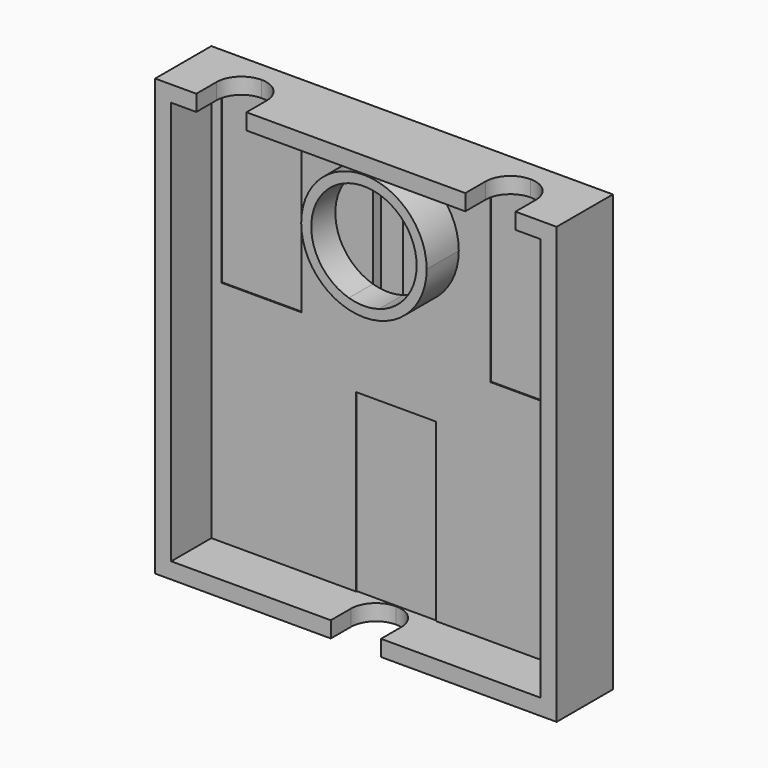
from build123d import *

# Parameters (mm, degrees)
F0_W      = 40
F0_H      = 43.4234265382
F1_DEPTH  = 2
F2_W      = 40
F2_H      = 43.4234265382
F2_W_2    = 36.8
F2_H_2    = 40.2234265382
F3_DEPTH  = 5
F5_DEPTH  = 1.6
F7_DEPTH  = 1
F8_DEPTH  = 4
F9_DEPTH  = 1
F11_DEPTH = 1.6
F13_DEPTH = 0.1


with BuildPart() as f1:
    # F0 (on Front) → F1 (new body)
    with BuildSketch(Plane.XZ):
        with Locations((-15.7519546337, 17.2915523872)):
            Rectangle(F0_W, F0_H)
    extrude(amount=F1_DEPTH)

    # F2 (on face) → F3 (join)
    with BuildSketch(Plane.XZ.offset(2)):
        with Locations((-15.7519546337, 17.2915523872)):
            Rectangle(F2_W, F2_H)
        with Locations((-15.7519546337, 17.2915523872)):
            Rectangle(F2_W_2, F2_H_2, mode=Mode.SUBTRACT)
    extrude(amount=F3_DEPTH)

    # F4 (on face) → F5 (cut, through all)
    with BuildSketch(Plane(origin=(0, 0, 37.4032656563), x_dir=(1, 0, 0), z_dir=(0, 0, -1))):
        with BuildLine():
            ThreePointArc((-4.8519546337, 4.5), (-4.1197215867, 2.732233047), (-2.3519546337, 2))
            ThreePointArc((-2.3519546337, 2), (-0.5841876808, 2.732233047), (0.1480453663, 4.5))
            ThreePointArc((0.1480453663, 4.5), (-0.5841876808, 6.267766953), (-2.3519546337, 7))
            ThreePointArc((-2.3519546337, 7), (-4.1197215867, 6.267766953), (-4.8519546337, 4.5))
        make_face()
        with BuildLine():
            ThreePointArc((-29.1519546337, 2), (-27.3841876808, 2.732233047), (-26.6519546337, 4.5))
            ThreePointArc((-26.6519546337, 4.5), (-27.3841876808, 6.267766953), (-29.1519546337, 7))
            ThreePointArc((-29.1519546337, 7), (-30.9197215867, 6.267766953), (-31.6519546337, 4.5))
            ThreePointArc((-31.6519546337, 4.5), (-30.9197215867, 2.732233047), (-29.1519546337, 2))
        make_face()
        with BuildLine():
            ThreePointArc((-29.1519546337, 7), (-27.3841876808, 6.267766953), (-26.6519546337, 4.5))
            Line((-26.6519546337, 4.5), (-26.6519546337, 7))
            Line((-26.6519546337, 7), (-29.1519546337, 7))
        make_face()
        with BuildLine():
            ThreePointArc((-31.6519546337, 4.5), (-30.9197215867, 6.267766953), (-29.1519546337, 7))
            Line((-29.1519546337, 7), (-31.6519546337, 7))
            Line((-31.6519546337, 7), (-31.6519546337, 4.5))
        make_face()
        with BuildLine():
            Line((-2.3519546337, 7), (-4.8519546337, 7))
            Line((-4.8519546337, 7), (-4.8519546337, 4.5))
            ThreePointArc((-4.8519546337, 4.5), (-4.1197215867, 6.267766953), (-2.3519546337, 7))
        make_face()
        with BuildLine():
            ThreePointArc((-2.3519546337, 7), (-0.5841876808, 6.267766953), (0.1480453663, 4.5))
            Line((0.1480453663, 4.5), (0.1480453663, 7))
            Line((0.1480453663, 7), (-2.3519546337, 7))
        make_face()
    extrude(amount=-F5_DEPTH, mode=Mode.SUBTRACT)

    # F6 (on face) → F7 (join)
    with BuildSketch(Plane.XZ.offset(2)):
        with BuildLine():
            Line((-17.2519546337, 25.3721127069), (-17.2519546337, 35.4344186057))
            ThreePointArc((-17.2519546337, 35.4344186057), (-21.0019546337, 30.4032656563), (-17.2519546337, 25.3721127069))
        make_face()
        with BuildLine():
            ThreePointArc((-14.2519546337, 25.3721127069), (-11.5425900736, 27.2657905568), (-10.5019546337, 30.4032656563))
            ThreePointArc((-10.5019546337, 30.4032656563), (-11.5425900736, 33.5407407558), (-14.2519546337, 35.4344186057))
            Line((-14.2519546337, 35.4344186057), (-14.2519546337, 25.3721127069))
        make_face()
    extrude(amount=F7_DEPTH)

    # F6 (on face) → F8 (join)
    with BuildSketch(Plane.XZ.offset(2)):
        with BuildLine():
            ThreePointArc((-14.2519546337, 35.4344186057), (-11.5425900736, 33.5407407558), (-10.5019546337, 30.4032656563))
            ThreePointArc((-10.5019546337, 30.4032656563), (-11.5425900736, 27.2657905568), (-14.2519546337, 25.3721127069))
            Line((-14.2519546337, 25.3721127069), (-14.2519546337, 24.3359351065))
            ThreePointArc((-14.2519546337, 24.3359351065), (-10.8306997125, 26.5505069044), (-9.5019546337, 30.4032656563))
            ThreePointArc((-9.5019546337, 30.4032656563), (-10.8306997125, 34.2560244081), (-14.2519546337, 36.470596206))
            Line((-14.2519546337, 36.470596206), (-14.2519546337, 35.4344186057))
        make_face()
        with BuildLine():
            ThreePointArc((-17.2519546337, 35.4344186057), (-15.7519546337, 35.6532656563), (-14.2519546337, 35.4344186057))
            Line((-14.2519546337, 35.4344186057), (-14.2519546337, 36.470596206))
            ThreePointArc((-14.2519546337, 36.470596206), (-15.7519546337, 36.6532656563), (-17.2519546337, 36.470596206))
            Line((-17.2519546337, 36.470596206), (-17.2519546337, 35.4344186057))
        make_face()
        with BuildLine():
            Line((-14.2519546337, 24.3359351065), (-14.2519546337, 25.3721127069))
            ThreePointArc((-14.2519546337, 25.3721127069), (-15.7519546337, 25.1532656563), (-17.2519546337, 25.3721127069))
            Line((-17.2519546337, 25.3721127069), (-17.2519546337, 24.3359351065))
            ThreePointArc((-17.2519546337, 24.3359351065), (-15.7519546337, 24.1532656563), (-14.2519546337, 24.3359351065))
        make_face()
        with BuildLine():
            ThreePointArc((-17.2519546337, 25.3721127069), (-21.0019546337, 30.4032656563), (-17.2519546337, 35.4344186057))
            Line((-17.2519546337, 35.4344186057), (-17.2519546337, 36.470596206))
            ThreePointArc((-17.2519546337, 36.470596206), (-22.0019546337, 30.4032656563), (-17.2519546337, 24.3359351065))
            Line((-17.2519546337, 24.3359351065), (-17.2519546337, 25.3721127069))
        make_face()
    extrude(amount=F8_DEPTH)

    # F6 (on face) → F9 (cut)
    with BuildSketch(Plane.XZ.offset(2)):
        with BuildLine():
            ThreePointArc((-17.2519546337, 35.4344186057), (-15.7519546337, 35.6532656563), (-14.2519546337, 35.4344186057))
            Line((-14.2519546337, 35.4344186057), (-14.2519546337, 36.470596206))
            ThreePointArc((-14.2519546337, 36.470596206), (-15.7519546337, 36.6532656563), (-17.2519546337, 36.470596206))
            Line((-17.2519546337, 36.470596206), (-17.2519546337, 35.4344186057))
        make_face()
        with BuildLine():
            Line((-14.2519546337, 24.3359351065), (-14.2519546337, 25.3721127069))
            ThreePointArc((-14.2519546337, 25.3721127069), (-15.7519546337, 25.1532656563), (-17.2519546337, 25.3721127069))
            Line((-17.2519546337, 25.3721127069), (-17.2519546337, 24.3359351065))
            ThreePointArc((-17.2519546337, 24.3359351065), (-15.7519546337, 24.1532656563), (-14.2519546337, 24.3359351065))
        make_face()
    extrude(amount=F9_DEPTH, mode=Mode.SUBTRACT)

    # F10 (on face) → F11 (cut, through all)
    with BuildSketch(Plane.XY.offset(-2.8201608819)):
        with BuildLine():
            Line((-13.2519546337, -7), (-13.2519546337, -4.5))
            ThreePointArc((-13.2519546337, -4.5), (-13.9841876808, -6.267766953), (-15.7519546337, -7))
            Line((-15.7519546337, -7), (-13.2519546337, -7))
        make_face()
        with BuildLine():
            ThreePointArc((-15.7519546337, -7), (-13.9841876808, -6.267766953), (-13.2519546337, -4.5))
            ThreePointArc((-13.2519546337, -4.5), (-13.984187679, -2.7322330488), (-15.7519546286, -2))
            ThreePointArc((-15.7519546286, -2), (-17.5197215849, -2.7322330452), (-18.2519546337, -4.5))
            ThreePointArc((-18.2519546337, -4.5), (-17.5197215867, -6.267766953), (-15.7519546337, -7))
        make_face()
        with BuildLine():
            Line((-18.2519546337, -7), (-15.7519546337, -7))
            ThreePointArc((-15.7519546337, -7), (-17.5197215867, -6.267766953), (-18.2519546337, -4.5))
            Line((-18.2519546337, -4.5), (-18.2519546337, -7))
        make_face()
    extrude(amount=-F11_DEPTH, mode=Mode.SUBTRACT)

    # F12 (on face) → F13 (cut)
    with BuildSketch(Plane.XZ.offset(2)):
        Polygon((-29.1519546337, 37.4032656563), (-33.1519546337, 37.4032656563), (-33.1519546337, 19.9032656563), (-25.1519546337, 19.9032656563), (-25.1519546337, 37.4032656563), align=None)
        Polygon((-2.3519546468, 37.4032656563), (-6.3519546337, 37.4032656563), (-6.3519546337, 19.9032656563), (1.6480453663, 19.9032656563), (1.6480453663, 37.4032656563), align=None)
        Polygon((-19.7519546337, 14.6798391181), (-19.7519546337, -2.8201608819), (-15.7519546337, -2.8201608819), (-11.7519546337, -2.8201608819), (-11.7519546337, 14.6798391181), align=None)
    extrude(amount=-F13_DEPTH, mode=Mode.SUBTRACT)


solid = f1.part
